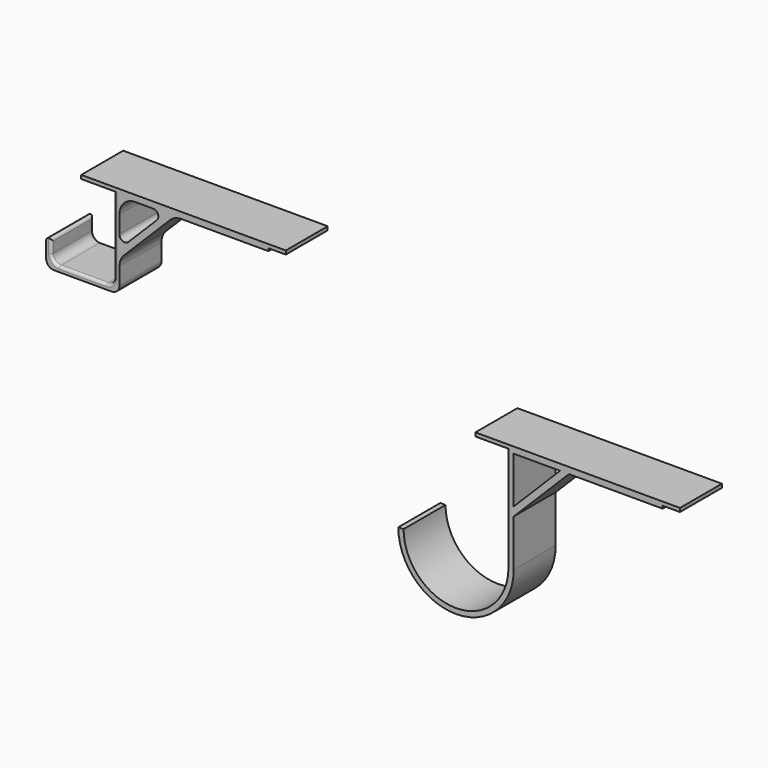
from build123d import *

# Parameters (mm, degrees)
F1_DEPTH = 25.4
F2_R     = 7.62
F3_R     = 2.54
F4_R     = 3.81
F5_R     = 1.26999
F7_DEPTH = 25.4


# Not quite as in the source:
# - a fillet or chamfer is up to 0.001 mm smaller than in the source, because OpenCascade refuses the exact size


with BuildPart() as f1:
    # F0 (on Front) → F1 (new body)
    with BuildSketch(Plane.XZ):
        Polygon((53.8098587847, 65.1143739842), (-45.2501412153, 65.1143739842), (-45.2501412153, 63.3363739842), (-29.2481412153, 63.3363739842), (-29.2481412153, 22.6963739842), (-59.7281412153, 22.6963739842), (-59.7281412153, 32.9748801887), (-62.2681412153, 32.9748801887), (-62.2681412153, 20.1563739842), (-26.7081412153, 20.1563739842), (-26.7081412153, 35.3582327689), (0, 62.0663739842), (45.4278587847, 62.0663739842), (45.4278587847, 63.3363739842), (53.8098587847, 63.3363739842), align=None)
        Polygon((-4.3186810799, 62.0663739842), (-26.7081412153, 39.5937040448), (-26.7081412153, 62.0663739842), align=None, mode=Mode.SUBTRACT)
    extrude(amount=F1_DEPTH)

    # F2
    f2_edges = [f1.edges().sort_by_distance(p)[0] for p in [
        (-26.708141, -12.7, 35.358233),
        (0, -12.7, 62.066374),
        (-26.708141, -12.7, 62.066374),
    ]]
    fillet(f2_edges, radius=F2_R)

    # F3
    f3_edges = [f1.edges().sort_by_distance(p)[0] for p in [
        (-26.708141, -12.7, 39.593704),
        (-4.318681, -12.7, 62.066374),
    ]]
    fillet(f3_edges, radius=F3_R)

    # F4
    f4_edges = [f1.edges().sort_by_distance(p)[0] for p in [
        (-29.248141, -12.7, 22.696374),
        (-59.728141, -12.7, 22.696374),
        (-26.708141, -12.7, 20.156374),
        (-62.268141, -12.7, 20.156374),
    ]]
    fillet(f4_edges, radius=F4_R)

    # F5 (radius 1.27 in the source; OpenCascade refuses exactly that, so slightly less here)
    f5_edges = [f1.edges().sort_by_distance(p)[0] for p in [
        (-44.488141, -25.4, 22.696374),
        (-30.364064, -25.4, 23.812297),
        (-29.248141, -25.4, 44.921374),
        (-29.248141, 0, 44.921374),
        (-30.364064, 0, 23.812297),
        (-59.728141, -12.7, 32.97488),
        (-62.268141, -12.7, 32.97488),
    ]]
    fillet(f5_edges, radius=F5_R)


with BuildPart() as f7:
    # F6 (on Front) → F7 (new body)
    with BuildSketch(Plane.XZ):
        with BuildLine():
            Line((70.7250546523, 17.4228777081), (-28.3349453477, 17.4228777081))
            Line((-28.3349453477, 17.4228777081), (-28.3349453477, 15.6448777081))
            Line((-28.3349453477, 15.6448777081), (-12.3329453477, 15.6448777081))
            Line((-12.3329453477, 15.6448777081), (-12.3329453477, -35.1551222919))
            ThreePointArc((-12.3329453477, -35.1551222919), (-37.7329453477, -60.5551222919), (-63.1329453477, -35.1551222919))
            Line((-63.1329453477, -35.1551222919), (-65.6730447201, -35.1551222919))
            ThreePointArc((-65.6730447201, -35.1551222919), (-37.6956862962, -63.0951968212), (-9.7929453477, -35.0806042552))
            Line((-9.7929453477, -35.0806042552), (-9.7929453477, -12.3994532244))
            Line((-9.7929453477, -12.3994532244), (16.9813855847, 14.3748777081))
            Line((16.9813855847, 14.3748777081), (62.3430546523, 14.3748777081))
            Line((62.3430546523, 14.3748777081), (62.3430546523, 15.6448777081))
            Line((62.3430546523, 15.6448777081), (70.7250546523, 15.6448777081))
            Line((70.7250546523, 15.6448777081), (70.7250546523, 17.4228777081))
        make_face()
        Polygon((12.6627045048, 14.3748777081), (-9.7929453477, -8.1642279407), (-9.7929453477, 14.3748777081), align=None, mode=Mode.SUBTRACT)
    extrude(amount=F7_DEPTH)


with BuildPart() as f7_1:
    # F8: moved
    add(f7.part.moved(Location((173.99, 0, 0))))


solid = Compound([f1.part, f7_1.part])
